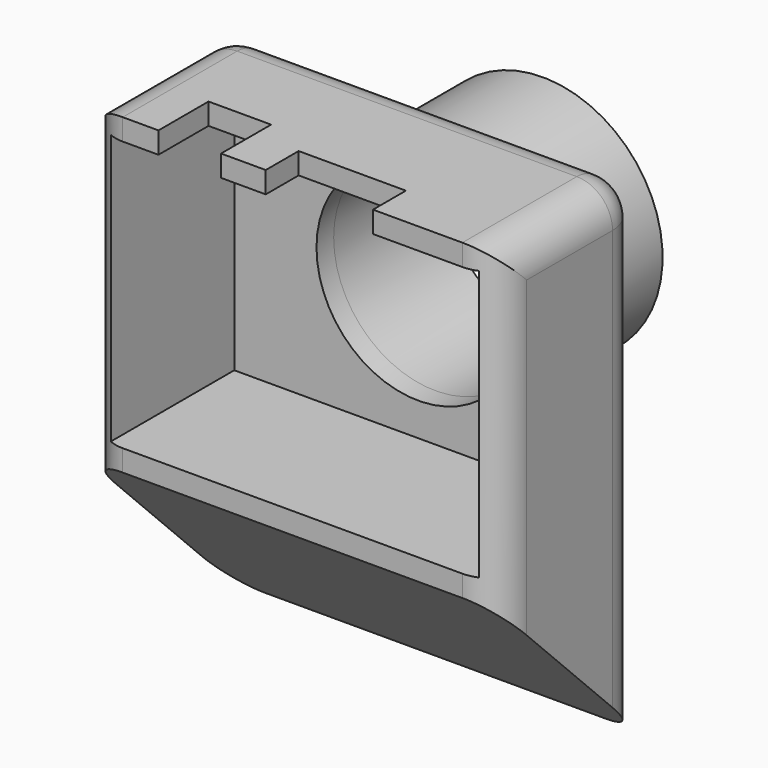
from build123d import *

# Parameters (mm, degrees)
F0_W          = 23
F0_H          = 17.5
F1_DEPTH      = 10
F2_T          = -1.2
F3_R          = 5.7
F4_DEPTH      = 3
F3_R_2        = 6.7
F5_DEPTH      = 7.5
F6_W          = 6
F6_H          = 2.3
F6_W_2        = 3.5
F6_H_2        = 3.5
F7_DEPTH      = 4
F8_DEPTH      = 10
F10_DEPTH     = 30
F11_T1_DEPTH  = 19
F11_T3_DEPTH  = 30.5
F11_T5_DEPTH  = 13
F11_T7_DEPTH  = 27.5
F11_S11_W     = 2
F11_S11_H     = 2
F11_T12_DEPTH = 2
F11_S17_W     = 2
F11_S17_H     = 2
F11_T18_DEPTH = 2


# Not quite as in the source:
# - a fillet or chamfer that OpenCascade refuses, or shapes differently, is made with other operations: its cross-section is extruded or revolved along the edge and cut away or added


with BuildPart() as f1:
    # F0 (on Front) → F1 (new body)
    with BuildSketch(Plane.XZ):
        Rectangle(F0_W, F0_H)
    extrude(amount=F1_DEPTH)

    # F2
    f2_openings = [f1.faces().sort_by_distance(p)[0] for p in [
        (0, -10, 0),
    ]]
    offset(amount=F2_T, openings=f2_openings)

    # F3 (on face) → F4 (cut)
    with BuildSketch(Plane(origin=(0, 0, 0), x_dir=(-1, 0, 0), z_dir=(0, 1, 0))):
        Circle(F3_R)
    extrude(amount=-F4_DEPTH, mode=Mode.SUBTRACT)

    # F3 (on face) → F5 (join)
    with BuildSketch(Plane(origin=(0, 0, 0), x_dir=(-1, 0, 0), z_dir=(0, 1, 0))):
        Circle(F3_R_2)
        Circle(F3_R, mode=Mode.SUBTRACT)
    extrude(amount=F5_DEPTH)

    # F6 (on face) → F7 (cut)
    with BuildSketch(Plane.XY.offset(8.75)):
        with Locations((1.5, -8.85)):
            Rectangle(F6_W, F6_H)
        with Locations((-5.75, -8.25)):
            Rectangle(F6_W_2, F6_H_2)
    extrude(amount=-F7_DEPTH, mode=Mode.SUBTRACT)

    # F8 (add): a face of the model
    f8_faces = [f1.faces().sort_by_distance(p)[0] for p in [
        (0, -5, -8.75),
    ]]
    extrude(f8_faces, amount=F8_DEPTH)

    # F9 (on face) → F10 (cut)
    with BuildSketch(Plane.YZ.offset(11.5)):
        Polygon((-10, -18.75), (0, -18.75), (-10, -8.75), align=None)
    extrude(amount=-F10_DEPTH, mode=Mode.SUBTRACT)

    # F11: fillet of radius 2 on 7 edges, made by hand

    # F11_s2 → F11_t1 (cut)
    with BuildSketch(Plane.YZ.offset(-9.5)):
        with BuildLine():
            ThreePointArc((0, 6.75), (-0.5857864376, 8.1642135624), (-2, 8.75))
            Line((-2, 8.75), (0, 8.75))
            Line((0, 8.75), (0, 6.75))
        make_face()
    extrude(amount=F11_T1_DEPTH, mode=Mode.SUBTRACT)

    # F11_s4 → F11_t3 (cut)
    with BuildSketch(Plane.XY.offset(-23.75)):
        with BuildLine():
            ThreePointArc((-11.5, -2), (-10.9142135624, -0.5857864376), (-9.5, 0))
            Line((-9.5, 0), (-11.5, 0))
            Line((-11.5, 0), (-11.5, -2))
        make_face()
        with BuildLine():
            ThreePointArc((9.5, 0), (10.9142135624, -0.5857864376), (11.5, -2))
            Line((11.5, -2), (11.5, 0))
            Line((11.5, 0), (9.5, 0))
        make_face()
    extrude(amount=F11_T3_DEPTH, mode=Mode.SUBTRACT)

    # F11_s6 → F11_t5 (cut)
    with BuildSketch(Plane.XZ.offset(2)):
        with BuildLine():
            ThreePointArc((9.5, 8.75), (10.9142135624, 8.1642135624), (11.5, 6.75))
            Line((11.5, 6.75), (11.5, 8.75))
            Line((11.5, 8.75), (9.5, 8.75))
        make_face()
        with BuildLine():
            ThreePointArc((-11.5, 6.75), (-10.9142135624, 8.1642135624), (-9.5, 8.75))
            Line((-9.5, 8.75), (-11.5, 8.75))
            Line((-11.5, 8.75), (-11.5, 6.75))
        make_face()
    extrude(amount=F11_T5_DEPTH, mode=Mode.SUBTRACT)

    # F11_s8 → F11_t7 (cut)
    with BuildSketch(Plane.XY.offset(-13.75)):
        with BuildLine():
            ThreePointArc((9.5, -10), (10.9142135624, -9.4142135624), (11.5, -8))
            Line((11.5, -8), (11.5, -10))
            Line((11.5, -10), (9.5, -10))
        make_face()
        with BuildLine():
            ThreePointArc((-11.5, -8), (-10.9142135624, -9.4142135624), (-9.5, -10))
            Line((-9.5, -10), (-11.5, -10))
            Line((-11.5, -10), (-11.5, -8))
        make_face()
    extrude(amount=F11_T7_DEPTH, mode=Mode.SUBTRACT)


with BuildPart() as f11_tool10:
    # F11_s11 → F11_t12 (new body)
    with BuildSketch(Plane.XZ.offset(2)):
        with Locations((10.5, 7.75)):
            Rectangle(F11_S11_W, F11_S11_H)
    extrude(amount=-F11_T12_DEPTH)

    # F11_s13 → F11_t14 (revolve, cut)
    with BuildSketch(Plane(origin=(9.5, -2, 6.75), x_dir=(-0.7071067812, 0, -0.7071067812), z_dir=(0.7071067812, 0, -0.7071067812))):
        with BuildLine():
            ThreePointArc((0, -2), (2, 0), (0, 2))
            Line((0, 2), (0, -2))
        make_face()
    revolve(axis=Axis((9.5, -2, 6.75), (0, 1, 0)), mode=Mode.SUBTRACT)


with BuildPart() as f1_1:
    add(f1.part)

    # F11_t9: cut F11_tool10
    add(f11_tool10.part, mode=Mode.SUBTRACT)


with BuildPart() as f11_tool16:
    # F11_s17 → F11_t18 (new body)
    with BuildSketch(Plane.YZ.offset(-9.5)):
        with Locations((-1, 7.75)):
            Rectangle(F11_S17_W, F11_S17_H)
    extrude(amount=-F11_T18_DEPTH)

    # F11_s19 → F11_t20 (revolve, cut)
    with BuildSketch(Plane(origin=(-9.5, -2, 6.75), x_dir=(0, -0.7071067812, -0.7071067812), z_dir=(0, 0.7071067812, -0.7071067812))):
        with BuildLine():
            ThreePointArc((0, -2), (2, 0), (0, 2))
            Line((0, 2), (0, -2))
        make_face()
    revolve(axis=Axis((-9.5, -2, 6.75), (-1, 0, 0)), mode=Mode.SUBTRACT)


with BuildPart() as f1_2:
    add(f1_1.part)

    # F11_t15: cut F11_tool16
    add(f11_tool16.part, mode=Mode.SUBTRACT)


solid = f1_2.part
